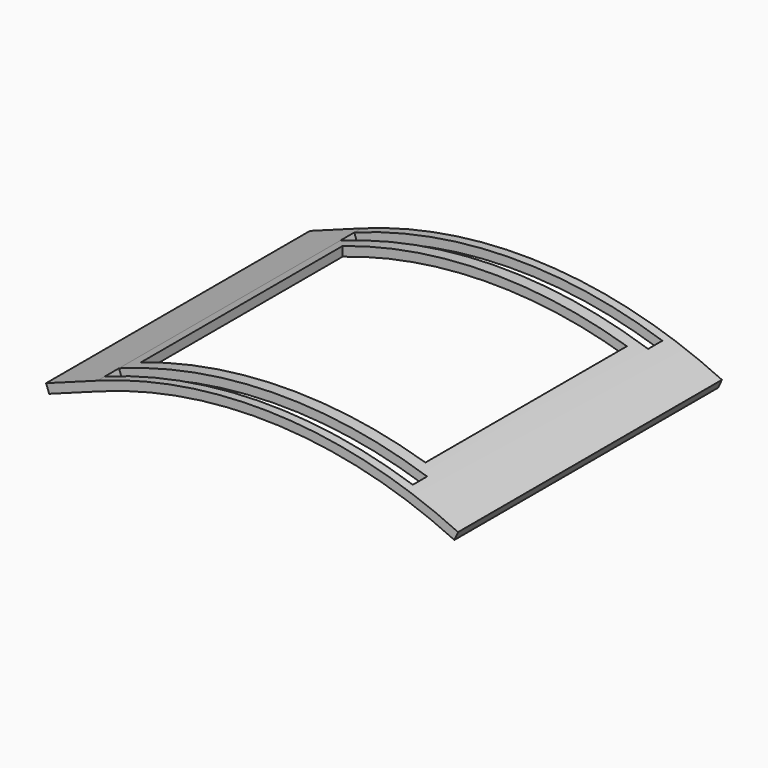
from build123d import *

# Parameters (mm, degrees)
F1_DEPTH  = 406
F4_DEPTH  = 22
F7_DEPTH  = 22
F9_W      = 350
F9_H      = 310
F10_DEPTH = 200


# Not quite as in the source:
# - ends of sketch curves that miss each other by under 0.0002 mm in the source are joined


with BuildPart() as f1:
    # F0 (on Front) → F1 (new body)
    with BuildSketch(Plane.XZ):
        with BuildLine():
            ThreePointArc((-186.3848490661, -11.1654008205), (33.2859089962, 22.935224068), (249.0237497892, -30.686400445))
            Line((249.0237497892, -30.686400445), (253.556713, -20.661948))
            ThreePointArc((253.556713, -20.661948), (33.6810541326, 33.9285497238), (-190.1858030941, -0.8429617445))
            Line((-190.1858030941, -0.8429617445), (-253.556714, -24.177561))
            Line((-253.556714, -24.177561), (-249.755724, -34.499987))
            Line((-249.755724, -34.499987), (-186.3848490661, -11.1654008205))
        make_face()
    extrude(amount=F1_DEPTH)

    # F3 (on offset) → F4 (cut)
    with BuildSketch(Plane.XZ.offset(395)):
        with BuildLine():
            Line((184.0178133859, -9.9744413883), (190.6417317828, 9.9535215049))
            ThreePointArc((190.6417317828, 9.9535215049), (-1.1548935515, 39.4263138769), (-191.9135098522, 3.8490558767))
            Line((-191.9135098522, 3.8490558767), (-184.6571423005, -15.8574184389))
            ThreePointArc((-184.6571423005, -15.8574184389), (-0.819837913, 18.4289869585), (184.0178133859, -9.9744413883))
        make_face()
    extrude(amount=-F4_DEPTH, mode=Mode.SUBTRACT)

    # F6 (on offset) → F7 (cut)
    with BuildSketch(Plane(origin=(0, -11, 0), x_dir=(-1, 0, 0), z_dir=(0, 1, 0))):
        with BuildLine():
            ThreePointArc((191.9135098522, 3.8490558767), (1.1548935515, 39.4263138769), (-190.6417317828, 9.9535215049))
            Line((-190.6417317828, 9.9535215049), (-184.0178133859, -9.9744413883))
            ThreePointArc((-184.0178133859, -9.9744413883), (0.819837913, 18.4289869585), (184.6571423005, -15.8574184389))
            Line((184.6571423005, -15.8574184389), (191.9135098522, 3.8490558767))
        make_face()
    extrude(amount=-F7_DEPTH, mode=Mode.SUBTRACT)

    # F9 (on offset) → F10 (cut)
    with BuildSketch(Plane.XY.offset(134)):
        with Locations((-5e-07, -203)):
            Rectangle(F9_W, F9_H)
    extrude(amount=-F10_DEPTH, mode=Mode.SUBTRACT)


solid = f1.part
